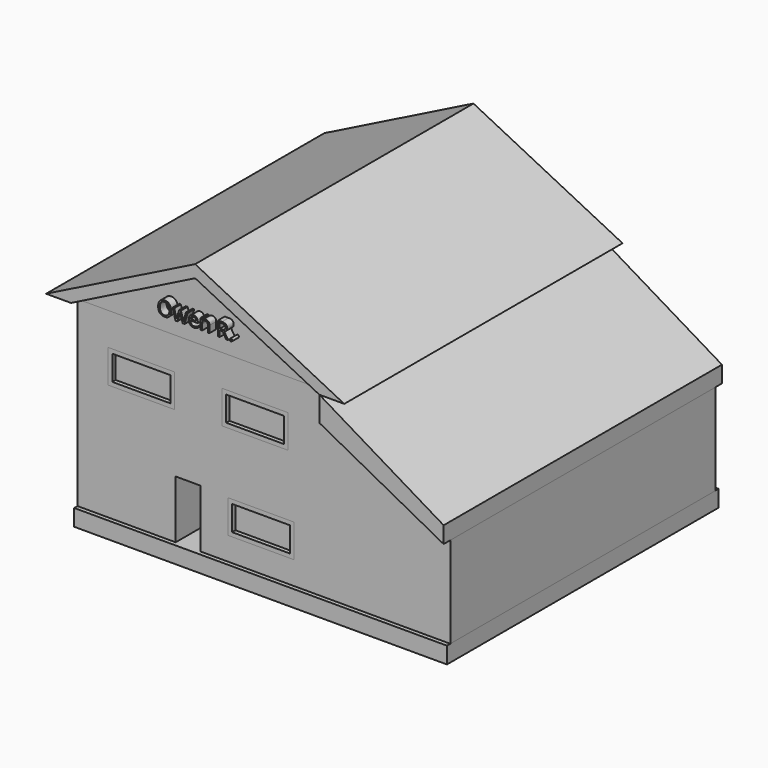
from build123d import *

# Parameters (mm, degrees)
F0_W         = 2438.4002349854
F0_H         = 1219.2002349854
F0_W_2       = 2438.3999965668
F0_H_2       = 1219.1999965668
F0_W_3       = 2438.4000267029
F0_H_3       = 1219.2000267029
F1_DEPTH     = 6096
F2_DEPTH     = 6248.4
F3_DEPTH     = 6400.8
F4_DEPTH     = 6096
F0_W_4       = 2133.6
F0_H_4       = 914.4
F5_DEPTH     = 5943.6
F6_DEPTH     = 6096
F7_TEXT_SIZE = 728.8696037398
F8_DEPTH     = 304.8


# Not quite as in the source:
# - Text() gives the source's letters only with a copy of the font that has no kerning and outlines rounded to 1/6400 em; it was checked with that copy


with BuildPart() as f1:
    # F0 (on Front) → F1 (new body, symmetric)
    with BuildSketch(Plane.XZ):
        Polygon((9144, -3352.8), (4572, -914.4), (4572, -6705.6), (9144, -6705.6), align=None)
        Polygon((4572, 0), (0, 0), (-4572, 0), (-4572, -6705.6), (-961.6174697876, -6705.6), (-961.6174697876, -4572), (-47.2174697876, -4572), (-47.2174697876, -6705.6), (4572, -6705.6), (4572, -914.4), align=None)
        with Locations((2180.9243577003, -5243.3620002747)):
            Rectangle(F0_W, F0_H, mode=Mode.SUBTRACT)
        with Locations((-2226.2431365967, -1808.947851944)):
            Rectangle(F0_W_2, F0_H_2, mode=Mode.SUBTRACT)
        with Locations((1962.5509994507, -1769.243529129)):
            Rectangle(F0_W_3, F0_H_3, mode=Mode.SUBTRACT)
    extrude(amount=F1_DEPTH, both=True)


with BuildPart() as f2:
    # F0 (on Front) → F2 (new body, symmetric)
    with BuildSketch(Plane.XZ):
        Polygon((-961.6174697876, -6705.6), (-4572, -6705.6), (-4572, -7315.2), (9144, -7315.2), (9144, -6705.6), (4572, -6705.6), (-47.2174697876, -6705.6), align=None)
    extrude(amount=F2_DEPTH, both=True)


with BuildPart() as f3:
    # F0 (on Front) → F3 (new body, symmetric)
    with BuildSketch(Plane.XZ):
        Polygon((-5486.4, 0), (-4572, 0), (0, 2286), (0, 2743.2), align=None)
        Polygon((0, 2286), (4572, 0), (5486.4, 0), (0, 2743.2), align=None)
    extrude(amount=F3_DEPTH, both=True)


with BuildPart() as f3b:
    # F0 (on Front) → F3, piece 2 (new body, symmetric)
    with BuildSketch(Plane.XZ):
        Polygon((9144, -2743.2), (4572, 0), (4572, -914.4), (9144, -3352.8), align=None)
    extrude(amount=F3_DEPTH, both=True)


with BuildPart() as f4:
    # F0 (on Front) → F4 (new body, symmetric)
    with BuildSketch(Plane.XZ):
        Polygon((-4572, 0), (0, 0), (0, 2286), align=None)
        Polygon((0, 2286), (0, 0), (4572, 0), align=None)
    extrude(amount=F4_DEPTH, both=True)

    # F7 (on face) → F8 (join)
    with BuildSketch(Plane.XZ.offset(6096)):
        with Locations((-1407.3808193207, 676.8547296524)):
            Text('Owen R.', F7_TEXT_SIZE, font='Open Sans', text_align=(TextAlign.LEFT, TextAlign.BOTTOM))
    extrude(amount=F8_DEPTH)


with BuildPart() as f5:
    # F0 (on Front) → F5 (new body, symmetric)
    with BuildSketch(Plane.XZ):
        with Locations((1962.5509994507, -1769.243529129)):
            Rectangle(F0_W_4, F0_H_4)
    extrude(amount=F5_DEPTH, both=True)


with BuildPart() as f5b:
    # F0 (on Front) → F5, piece 2 (new body, symmetric)
    with BuildSketch(Plane.XZ):
        with Locations((-2226.2431365967, -1808.947851944)):
            Rectangle(F0_W_4, F0_H_4)
    extrude(amount=F5_DEPTH, both=True)


with BuildPart() as f5c:
    # F0 (on Front) → F5, piece 3 (new body, symmetric)
    with BuildSketch(Plane.XZ):
        with Locations((2180.9243577003, -5243.3620002747)):
            Rectangle(F0_W_4, F0_H_4)
    extrude(amount=F5_DEPTH, both=True)


with BuildPart() as f6:
    # F0 (on Front) → F6 (new body, symmetric)
    with BuildSketch(Plane.XZ):
        with Locations((2180.9243577003, -5243.3620002747)):
            Rectangle(F0_W, F0_H)
        with Locations((2180.9243577003, -5243.3620002747)):
            Rectangle(F0_W_4, F0_H_4, mode=Mode.SUBTRACT)
    extrude(amount=F6_DEPTH, both=True)


with BuildPart() as f6b:
    # F0 (on Front) → F6, piece 2 (new body, symmetric)
    with BuildSketch(Plane.XZ):
        with Locations((1962.5509994507, -1769.243529129)):
            Rectangle(F0_W_3, F0_H_3)
        with Locations((1962.5509994507, -1769.243529129)):
            Rectangle(F0_W_4, F0_H_4, mode=Mode.SUBTRACT)
    extrude(amount=F6_DEPTH, both=True)


with BuildPart() as f6c:
    # F0 (on Front) → F6, piece 3 (new body, symmetric)
    with BuildSketch(Plane.XZ):
        with Locations((-2226.2431365967, -1808.947851944)):
            Rectangle(F0_W_2, F0_H_2)
        with Locations((-2226.2431365967, -1808.947851944)):
            Rectangle(F0_W_4, F0_H_4, mode=Mode.SUBTRACT)
    extrude(amount=F6_DEPTH, both=True)


solid = Compound([f1.part, f2.part, f3.part, f3b.part, f4.part, f5.part, f5b.part, f5c.part, f6.part, f6b.part, f6c.part])
